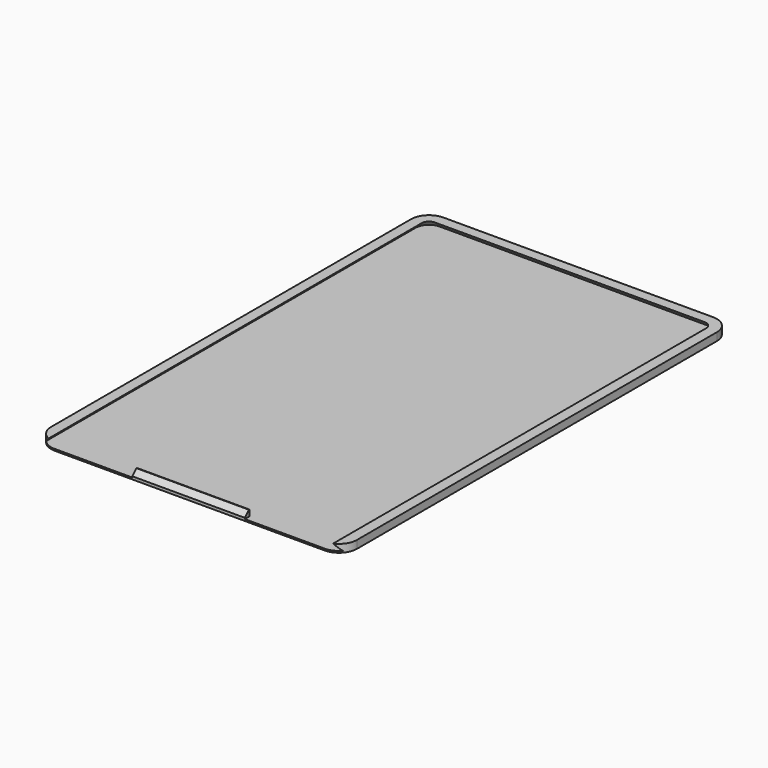
from build123d import *

# Parameters (mm, degrees)
F1_ANGLE      = 90
F3_DEPTH      = 24
F5_DEPTH      = 40
F9_DEPTH      = 25
F10_W         = 20
F10_H         = 1
F11_DEPTH     = 1.1
F12_SIZE      = 0.9
F13_TEXT_SIZE = 5.5555555556
F14_DEPTH     = 0.1
F16_DEPTH     = 0.1


# Not quite as in the source:
# - Text() gives the source's letters only with a copy of the font that has no kerning and outlines rounded to 1/6400 em; it was checked with that copy


with BuildPart() as f1:
    # F0 (on Front) → F1 (revolve)
    with BuildSketch(Plane.XZ):
        Polygon((-3.2, 1.4), (-3.2, 0), (0, 0), (0, 0.3), (-2.4, 0.3), (-1.3, 1.4), align=None)
    revolve(axis=Axis((0, 0, 0.5619533081), (0, 0, 1)), revolution_arc=F1_ANGLE)

    # F2 (on face) → F3 (join)
    with BuildSketch(Plane.YZ):
        Polygon((-2.4, 0.3), (-1.3, 1.4), (-3.2, 1.4), (-3.2, 0), (0, 0), (0, 0.3), align=None)
    extrude(amount=F3_DEPTH)

    # F4 (on face) → F5 (join)
    with BuildSketch(Plane(origin=(0, 0, 0), x_dir=(-1, 0, 0), z_dir=(0, 1, 0))):
        Polygon((3.2, 0), (3.2, 1.4), (1.3, 1.4), (2.4, 0.3), (-24, 0.3), (-24, 0), align=None)
    extrude(amount=F5_DEPTH)

    # F6: F1 across face


with BuildPart() as f1_1:
    add(f1.part)
    add(f1.part.mirror(Plane(origin=(24, 16.2526710511, 0.2296411676), x_dir=(0, 1, 0), z_dir=(1, 0, 0))))

    # F7: F1 across face


with BuildPart() as f1_2:
    add(f1_1.part)
    add(f1_1.part.mirror(Plane(origin=(24, 40, 0.2692759634), x_dir=(-1, 0, 0), z_dir=(0, 1, 0))))

    # F8 (on face) → F9 (cut)
    with BuildSketch(Plane.XZ.offset(3.2)):
        Polygon((-2.4, 0.3), (24, 0.3), (50.4, 0.3), (49.3, 1.4), (24, 1.4), (-1.3, 1.4), align=None)
    extrude(amount=-F9_DEPTH, mode=Mode.SUBTRACT)

    # F10 (on face) → F11 (join, through all)
    with BuildSketch(Plane.XY.offset(0.3)):
        with Locations((23.8, -2.7)):
            Rectangle(F10_W, F10_H)
    extrude(amount=F11_DEPTH)

    # F12
    f12_edges = [f1_2.edges().sort_by_distance(p)[0] for p in [
        (23.8, -3.2, 1.4),
    ]]
    chamfer(f12_edges, length=F12_SIZE)

    # F13 (on face) → F14 (cut)
    with BuildSketch(Plane(origin=(0, 0, 0), x_dir=(1, 0, 0), z_dir=(0, 0, -1))):
        with Locations(Location((1.8, -16.2303819444), (0, 0, -90))):
            Text('Simcard Carrier by BDM', F13_TEXT_SIZE, font='Open Sans', text_align=(TextAlign.LEFT, TextAlign.BOTTOM))
    extrude(amount=-F14_DEPTH, mode=Mode.SUBTRACT)

    # F15 (on face) → F16 (cut)
    with BuildSketch(Plane(origin=(0, 0, 0), x_dir=(1, 0, 0), z_dir=(0, 0, -1))):
        Polygon((1.8, -14.8), (5.8, -14.8), (5.8, -12.8), (4.8, -11.8), (1.8, -11.8), align=None)
    extrude(amount=-F16_DEPTH, mode=Mode.SUBTRACT)


solid = f1_2.part
